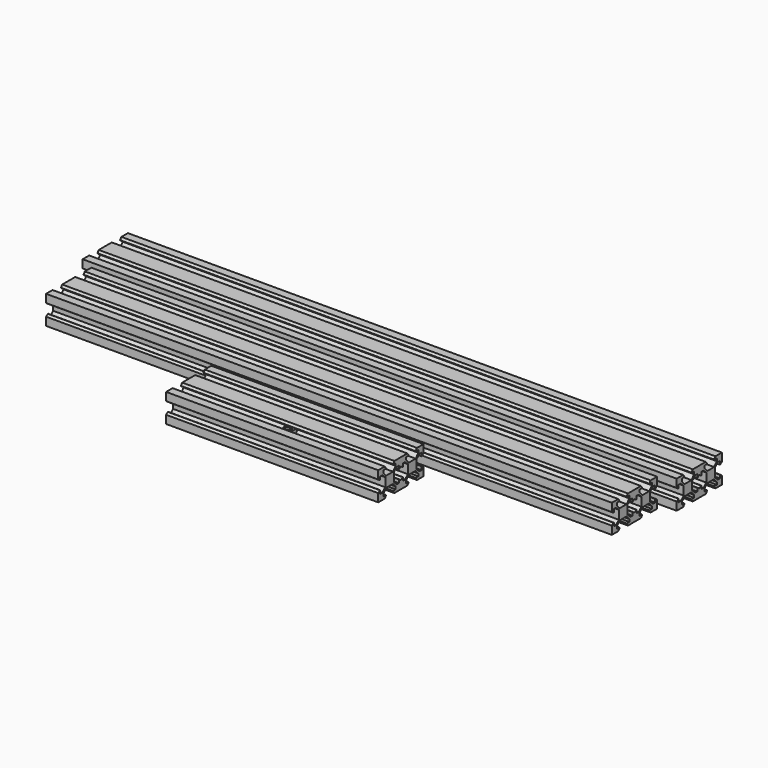
from build123d import *

# Parameters (mm, degrees)
F1_DEPTH  = 210
F4_DEPTH  = 75
F7_DEPTH  = 200
F9_DEPTH  = 5.9
F10_R     = 2.5
F11_DEPTH = 1
F12_R     = 1.6
F13_DEPTH = 4.445


# Not quite as in the source:
# - ends of sketch curves that miss each other by under 0.0002 mm in the source are joined


with BuildPart() as f1:
    # F0 (on Right) → F1 (new body, symmetric)
    with BuildSketch(Plane.YZ):
        Polygon((10.2685737705, -3.9572489457), (10.2685737705, -9.7132455008), (16.0245702043, -9.7132455008), (17.1575736492, -8.1377445729), (17.1575736492, -7.9352455008), (14.8075736492, -7.9352455008), (14.8075736492, -6.1572455008), (17.1570736492, -3.4902455008), (20.2685736492, -3.4902455008), (23.3800736492, -3.4902455008), (25.7295736492, -6.1572455008), (25.7295736492, -7.9352455008), (23.3795736492, -7.9352455008), (23.3795736492, -8.1377445729), (24.5125770941, -9.7132455008), (30.2685736492, -9.7132455008), (30.2685736492, -3.9572489457), (28.6930727214, -2.8242455008), (28.4905736492, -2.8242455008), (28.4905736492, -5.1742455008), (26.7125736492, -5.1742455008), (24.0455736492, -2.8247455008), (24.0455736492, 0.2867544992), (24.0455736492, 3.3982544992), (26.7125736492, 5.7477544992), (28.4905736492, 5.7477544992), (28.4905736492, 3.3977544992), (28.6930727214, 3.3977544992), (30.2685736492, 4.5307579441), (30.2685736492, 10.2867544992), (24.5125770941, 10.2867544992), (23.3795736492, 8.7112535713), (23.3795736492, 8.5087544992), (25.7295736492, 8.5087544992), (25.7295736492, 6.7307544992), (23.3800736492, 4.0637544992), (20.2685736492, 4.0637544992), (17.1570736492, 4.0637544992), (14.8075736492, 6.7307544992), (14.8075736492, 8.5087544992), (17.1575736492, 8.5087544992), (17.1575736492, 8.7112535713), (16.0245702043, 10.2867544992), (10.2685736492, 10.2867544992), (10.2685737705, 4.5307579441), (11.8440745771, 3.3977544992), (12.0465736492, 3.3977544992), (12.0465736492, 5.7477544992), (13.8245736492, 5.7477544992), (16.4915736492, 3.3982544992), (16.4915736492, 0.2867544992), (16.4915736492, -2.8247455008), (13.8245736492, -5.1742455008), (12.0465736492, -5.1742455008), (12.0465736492, -2.8242455008), (11.8440745771, -2.8242455008), align=None)
        Polygon((4.5125772154, -9.7132455008), (10.2685737705, -9.7132455008), (10.2685737705, -3.9572489457), (8.6930728426, -2.8242455008), (8.4905737705, -2.8242455008), (8.4905737705, -5.1742455008), (6.7125737705, -5.1742455008), (4.0455737705, -2.8247455008), (4.0455737705, 0.2867544992), (4.0455737705, 3.3982544992), (6.7125737705, 5.7477544992), (8.4905737705, 5.7477544992), (8.4905737705, 3.3977544992), (8.6930728426, 3.3977544992), (10.2685737705, 4.5307579441), (10.2685737705, 10.2867544992), (4.5125772154, 10.2867544992), (3.3795737705, 8.7112535713), (3.3795737705, 8.5087544992), (5.7295737705, 8.5087544992), (5.7295737705, 6.7307544992), (3.3800737705, 4.0637544992), (0.2685737705, 4.0637544992), (-2.8429262295, 4.0637544992), (-5.1924262295, 6.7307544992), (-5.1924262295, 8.5087544992), (-2.8424262295, 8.5087544992), (-2.8424262295, 8.7112535713), (-3.9754296744, 10.2867544992), (-9.7314262295, 10.2867544992), (-9.7314262295, 4.5307579441), (-8.1559253016, 3.3977544992), (-7.9534262295, 3.3977544992), (-7.9534262295, 5.7477544992), (-6.1754262295, 5.7477544992), (-3.5084262295, 3.3982544992), (-3.5084262295, 0.2867544992), (-3.5084262295, -2.8247455008), (-6.1754262295, -5.1742455008), (-7.9534262295, -5.1742455008), (-7.9534262295, -2.8242455008), (-8.1559253016, -2.8242455008), (-9.7314262295, -3.9572489457), (-9.7314262295, -9.7132455008), (-3.9754296744, -9.7132455008), (-2.8424262295, -8.1377445729), (-2.8424262295, -7.9352455008), (-5.1924262295, -7.9352455008), (-5.1924262295, -6.1572455008), (-2.8429262295, -3.4902455008), (0.2685737705, -3.4902455008), (3.3800737705, -3.4902455008), (5.7295737705, -6.1572455008), (5.7295737705, -7.9352455008), (3.3795737705, -7.9352455008), (3.3795737705, -8.1377445729), align=None)
    extrude(amount=F1_DEPTH, both=True)


with BuildPart() as f1_1:
    # F3: moved
    add(f1.part.moved(Location((0, 35.2, 0))))


with BuildPart() as f4:
    # F2 (on Right) → F4 (new body, symmetric)
    with BuildSketch(Plane.YZ):
        Polygon((-5.0975223597, -9.7629997892), (0.6584741954, -9.7629997892), (0.6584741954, -4.0070032341), (-0.9170267324, -2.8739997892), (-1.1195258046, -2.8739997892), (-1.1195258046, -5.2239997892), (-2.8975258046, -5.2239997892), (-5.5645258046, -2.8744997892), (-5.5645258046, 0.2370002108), (-5.5645258046, 3.3485002108), (-2.8975258046, 5.6980002108), (-1.1195258046, 5.6980002108), (-1.1195258046, 3.3480002108), (-0.9170267324, 3.3480002108), (0.6584741954, 4.4810036557), (0.6584741954, 10.2370002108), (-5.0975223597, 10.2370002108), (-6.2305258046, 8.6614992829), (-6.2305258046, 8.4590002108), (-3.8805258046, 8.4590002108), (-3.8805258046, 6.6810002108), (-6.2300258046, 4.0140002108), (-9.3415258046, 4.0140002108), (-12.4530258046, 4.0140002108), (-14.8025258046, 6.6810002108), (-14.8025258046, 8.4590002108), (-12.4525258046, 8.4590002108), (-12.4525258046, 8.6614992829), (-13.5855292495, 10.2370002108), (-19.3415258046, 10.2370002108), (-19.3415258046, 4.4810036557), (-17.7660248767, 3.3480002108), (-17.5635258046, 3.3480002108), (-17.5635258046, 5.6980002108), (-15.7855258046, 5.6980002108), (-13.1185258046, 3.3485002108), (-13.1185258046, 0.2370002108), (-13.1185258046, -2.8744997892), (-15.7855258046, -5.2239997892), (-17.5635258046, -5.2239997892), (-17.5635258046, -2.8739997892), (-17.7660248767, -2.8739997892), (-19.3415258046, -4.0070032341), (-19.3415258046, -9.7629997892), (-13.5855292495, -9.7629997892), (-12.4525258046, -8.1874988613), (-12.4525258046, -7.9849997892), (-14.8025258046, -7.9849997892), (-14.8025258046, -6.2069997892), (-12.4530258046, -3.5399997892), (-9.3415258046, -3.5399997892), (-6.2300258046, -3.5399997892), (-3.8805258046, -6.2069997892), (-3.8805258046, -7.9849997892), (-6.2305258046, -7.9849997892), (-6.2305258046, -8.1874988613), align=None)
        Polygon((0.6584741954, -4.0070032341), (0.6584741954, -9.7629997892), (6.4144706293, -9.7629997892), (7.5474740742, -8.1874988613), (7.5474740742, -7.9849997892), (5.1974740742, -7.9849997892), (5.1974740742, -6.2069997892), (7.5469740742, -3.5399997892), (10.6584740742, -3.5399997892), (13.7699740742, -3.5399997892), (16.1194740742, -6.2069997892), (16.1194740742, -7.9849997892), (13.7694740742, -7.9849997892), (13.7694740742, -8.1874988613), (14.9024775191, -9.7629997892), (20.6584740742, -9.7629997892), (20.6584740742, -4.0070032341), (19.0829731463, -2.8739997892), (18.8804740742, -2.8739997892), (18.8804740742, -5.2239997892), (17.1024740742, -5.2239997892), (14.4354740742, -2.8744997892), (14.4354740742, 0.2370002108), (14.4354740742, 3.3485002108), (17.1024740742, 5.6980002108), (18.8804740742, 5.6980002108), (18.8804740742, 3.3480002108), (19.0829731463, 3.3480002108), (20.6584740742, 4.4810036557), (20.6584740742, 10.2370002108), (14.9024775191, 10.2370002108), (13.7694740742, 8.6614992829), (13.7694740742, 8.4590002108), (16.1194740742, 8.4590002108), (16.1194740742, 6.6810002108), (13.7699740742, 4.0140002108), (10.6584740742, 4.0140002108), (7.5469740742, 4.0140002108), (5.1974740742, 6.6810002108), (5.1974740742, 8.4590002108), (7.5474740742, 8.4590002108), (7.5474740742, 8.6614992829), (6.4144706293, 10.2370002108), (0.6584740742, 10.2370002108), (0.6584741954, 4.4810036557), (2.233975002, 3.3480002108), (2.4364740742, 3.3480002108), (2.4364740742, 5.6980002108), (4.2144740742, 5.6980002108), (6.8814740742, 3.3485002108), (6.8814740742, 0.2370002108), (6.8814740742, -2.8744997892), (4.2144740742, -5.2239997892), (2.4364740742, -5.2239997892), (2.4364740742, -2.8739997892), (2.233975002, -2.8739997892), align=None)
    extrude(amount=F4_DEPTH, both=True)


with BuildPart() as f4_1:
    # F5: moved
    add(f4.part.moved(Location((0, -50.2, 0))))


with BuildPart() as f7:
    # F6 (on Right) → F7 (new body, symmetric)
    with BuildSketch(Plane.YZ):
        Polygon((-5.0975223597, -9.7629997892), (0.6584741954, -9.7629997892), (0.6584741954, -4.0070032341), (-0.9170267324, -2.8739997892), (-1.1195258046, -2.8739997892), (-1.1195258046, -5.2239997892), (-2.8975258046, -5.2239997892), (-5.5645258046, -2.8744997892), (-5.5645258046, 0.2370002108), (-5.5645258046, 3.3485002108), (-2.8975258046, 5.6980002108), (-1.1195258046, 5.6980002108), (-1.1195258046, 3.3480002108), (-0.9170267324, 3.3480002108), (0.6584741954, 4.4810036557), (0.6584741954, 10.2370002108), (-5.0975223597, 10.2370002108), (-6.2305258046, 8.6614992829), (-6.2305258046, 8.4590002108), (-3.8805258046, 8.4590002108), (-3.8805258046, 6.6810002108), (-6.2300258046, 4.0140002108), (-9.3415258046, 4.0140002108), (-12.4530258046, 4.0140002108), (-14.8025258046, 6.6810002108), (-14.8025258046, 8.4590002108), (-12.4525258046, 8.4590002108), (-12.4525258046, 8.6614992829), (-13.5855292495, 10.2370002108), (-19.3415258046, 10.2370002108), (-19.3415258046, 4.4810036557), (-17.7660248767, 3.3480002108), (-17.5635258046, 3.3480002108), (-17.5635258046, 5.6980002108), (-15.7855258046, 5.6980002108), (-13.1185258046, 3.3485002108), (-13.1185258046, 0.2370002108), (-13.1185258046, -2.8744997892), (-15.7855258046, -5.2239997892), (-17.5635258046, -5.2239997892), (-17.5635258046, -2.8739997892), (-17.7660248767, -2.8739997892), (-19.3415258046, -4.0070032341), (-19.3415258046, -9.7629997892), (-13.5855292495, -9.7629997892), (-12.4525258046, -8.1874988613), (-12.4525258046, -7.9849997892), (-14.8025258046, -7.9849997892), (-14.8025258046, -6.2069997892), (-12.4530258046, -3.5399997892), (-9.3415258046, -3.5399997892), (-6.2300258046, -3.5399997892), (-3.8805258046, -6.2069997892), (-3.8805258046, -7.9849997892), (-6.2305258046, -7.9849997892), (-6.2305258046, -8.1874988613), align=None)
        Polygon((0.6584741954, -4.0070032341), (0.6584741954, -9.7629997892), (6.4144706293, -9.7629997892), (7.5474740742, -8.1874988613), (7.5474740742, -7.9849997892), (5.1974740742, -7.9849997892), (5.1974740742, -6.2069997892), (7.5469740742, -3.5399997892), (10.6584740742, -3.5399997892), (13.7699740742, -3.5399997892), (16.1194740742, -6.2069997892), (16.1194740742, -7.9849997892), (13.7694740742, -7.9849997892), (13.7694740742, -8.1874988613), (14.9024775191, -9.7629997892), (20.6584740742, -9.7629997892), (20.6584740742, -4.0070032341), (19.0829731463, -2.8739997892), (18.8804740742, -2.8739997892), (18.8804740742, -5.2239997892), (17.1024740742, -5.2239997892), (14.4354740742, -2.8744997892), (14.4354740742, 0.2370002108), (14.4354740742, 3.3485002108), (17.1024740742, 5.6980002108), (18.8804740742, 5.6980002108), (18.8804740742, 3.3480002108), (19.0829731463, 3.3480002108), (20.6584740742, 4.4810036557), (20.6584740742, 10.2370002108), (14.9024775191, 10.2370002108), (13.7694740742, 8.6614992829), (13.7694740742, 8.4590002108), (16.1194740742, 8.4590002108), (16.1194740742, 6.6810002108), (13.7699740742, 4.0140002108), (10.6584740742, 4.0140002108), (7.5469740742, 4.0140002108), (5.1974740742, 6.6810002108), (5.1974740742, 8.4590002108), (7.5474740742, 8.4590002108), (7.5474740742, 8.6614992829), (6.4144706293, 10.2370002108), (0.6584740742, 10.2370002108), (0.6584741954, 4.4810036557), (2.233975002, 3.3480002108), (2.4364740742, 3.3480002108), (2.4364740742, 5.6980002108), (4.2144740742, 5.6980002108), (6.8814740742, 3.3485002108), (6.8814740742, 0.2370002108), (6.8814740742, -2.8744997892), (4.2144740742, -5.2239997892), (2.4364740742, -5.2239997892), (2.4364740742, -2.8739997892), (2.233975002, -2.8739997892), align=None)
    extrude(amount=F7_DEPTH, both=True)


with BuildPart() as f9:
    # F8 (on Right) → F9 (new body)
    with BuildSketch(Plane.YZ):
        Polygon((-54.5805258046, 7.9590002108), (-56.9305258046, 7.9590002108), (-62.1525258046, 7.9590002108), (-64.5025258046, 7.9590002108), (-64.5025258046, 6.8698273443), (-62.4271542822, 4.5140002108), (-56.6558973269, 4.5140002108), (-54.5805258046, 6.8698273443), align=None)
    extrude(amount=F9_DEPTH)

    # F10 (on face) → F11 (join)
    with BuildSketch(Plane.XY.offset(7.9590002108)):
        with Locations((2.95, -59.5415258046)):
            Circle(F10_R)
    extrude(amount=F11_DEPTH)

    # F12 (on face) → F13 (cut, through all)
    with BuildSketch(Plane.XY.offset(8.9590002108)):
        with Locations((2.95, -59.5415258046)):
            Circle(F12_R)
    extrude(amount=-F13_DEPTH, mode=Mode.SUBTRACT)


with BuildPart() as f14_1:
    # F14: copy of F9
    add(f9.part)


solid = Compound([f1_1.part, f4_1.part, f7.part, f9.part, f14_1.part])
